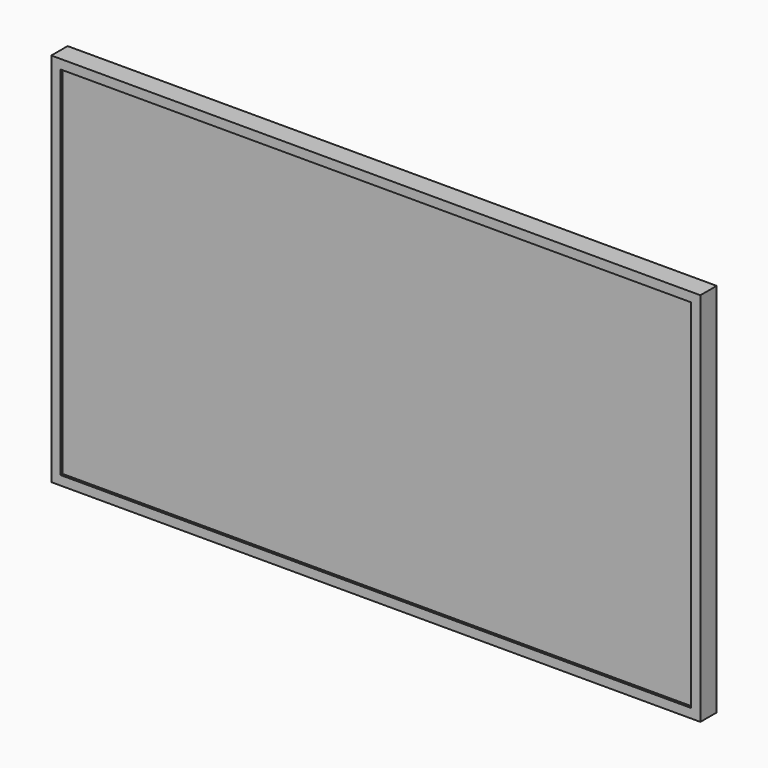
from build123d import *

# Parameters (mm, degrees)
F2_DEPTH      = 78
F3_DEPTH      = 10
F4_START      = -5
F4_DEPTH      = 5
F5_SIZE2      = 39
F5_SIZE       = 300
F1_W          = 55.88
F1_H          = 359.41
F6_DEPTH      = 75
F6_DEPTH_BACK = 75


with BuildPart() as f2:
    # F0 (on Front) → F2 (new body)
    with BuildSketch(Plane.XZ):
        Polygon((0, 779.78), (-621.03, 779.78), (-621.03, 420.37), (-603.3609412751, 420.37), (-603.3609412751, 762.1109412751), (0, 762.1109412751), align=None)
        Polygon((621.03, 779.78), (0, 779.78), (0, 762.1109412751), (603.3609412751, 762.1109412751), (603.3609412751, 78.6290587249), (-603.3609412751, 78.6290587249), (-603.3609412751, 420.37), (-621.03, 420.37), (-621.03, 60.96), (0, 60.96), (621.03, 60.96), align=None)
        Polygon((603.3609412751, 762.1109412751), (0, 762.1109412751), (-603.3609412751, 762.1109412751), (-603.3609412751, 420.37), (-603.3609412751, 78.6290587249), (603.3609412751, 78.6290587249), align=None)
    extrude(amount=-F2_DEPTH)

    # F0 (on Front) → F3 (cut)
    with BuildSketch(Plane.XZ):
        Polygon((603.3609412751, 762.1109412751), (0, 762.1109412751), (-603.3609412751, 762.1109412751), (-603.3609412751, 420.37), (-603.3609412751, 78.6290587249), (603.3609412751, 78.6290587249), align=None)
    extrude(amount=-F3_DEPTH, mode=Mode.SUBTRACT)

    # F5
    f5_edges = [f2.edges().sort_by_distance(p)[0] for p in [
        (0, 78, 779.78),
        (-621.03, 78, 420.37),
        (0, 78, 60.96),
        (621.03, 78, 420.37),
    ]]
    f5_side = f2.faces().sort_by_distance((0, 78, 420.37))[0]
    chamfer(f5_edges, length=F5_SIZE, length2=F5_SIZE2, reference=f5_side)

    # F1 (on Right) → F6 (join, two sides)
    with BuildSketch(Plane.YZ) as f6_sk:
        with Locations((83.82, 240.665)):
            Rectangle(F1_W, F1_H)
    extrude(amount=F6_DEPTH)
    extrude(f6_sk.sketch, amount=-F6_DEPTH_BACK)


with BuildPart() as f4:
    # F0 (on Front) → F4 (new body)
    with BuildSketch(Plane.XZ.offset(F4_START)):
        Polygon((603.3609412751, 762.1109412751), (0, 762.1109412751), (-603.3609412751, 762.1109412751), (-603.3609412751, 420.37), (-603.3609412751, 78.6290587249), (603.3609412751, 78.6290587249), align=None)
    extrude(amount=-F4_DEPTH)


solid = Compound([f2.part, f4.part])
